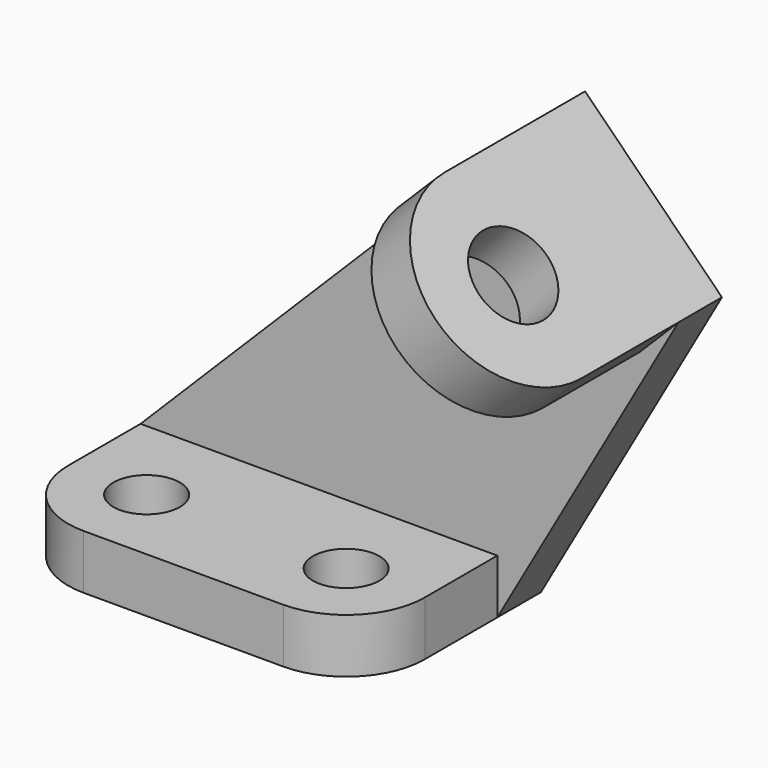
from build123d import *

# Parameters (mm, degrees)
F0_R     = 5.5
F1_DEPTH = 9
F2_DEPTH = 9
F4_DEPTH = 37
F5_DEPTH = 28
F6_R     = 7
F7_DEPTH = 9


with BuildPart() as f1:
    # F0 (on Top) → F1 (new body)
    with BuildSketch(Plane.XY):
        with BuildLine():
            ThreePointArc((-29.5, 13), (-25.6923881554, 3.8076118446), (-16.5, 0))
            Line((-16.5, 0), (16.5, 0))
            ThreePointArc((16.5, 0), (25.6923881554, 3.8076118446), (29.5, 13))
            Line((29.5, 13), (29.5, 37))
            Line((29.5, 37), (-29.5, 37))
            Line((-29.5, 37), (-29.5, 13))
        make_face()
        with Locations((-16.5, 13)):
            Circle(F0_R, mode=Mode.SUBTRACT)
        with Locations((16.5, 13)):
            Circle(F0_R, mode=Mode.SUBTRACT)
    extrude(amount=-F1_DEPTH)

    # F3 (on face) → F4 (join, through all)
    with BuildSketch(Plane.XZ):
        Polygon((36.813708499, 66.313708499), (25.5, 55), (48.127416998, 55), align=None)
        Polygon((48.127416998, 55), (25.5, 55), (-29.5, 0), (29.5, 0), (29.5, -9), (59.441125497, 43.686291501), align=None)
    extrude(amount=-F4_DEPTH)

    # F3 (on face) → F5 (cut)
    with BuildSketch(Plane.XZ):
        Polygon((36.813708499, 66.313708499), (25.5, 55), (48.127416998, 55), align=None)
        Polygon((48.127416998, 55), (25.5, 55), (-29.5, 0), (29.5, 0), (29.5, -9), (59.441125497, 43.686291501), align=None)
    extrude(amount=-F5_DEPTH, mode=Mode.SUBTRACT)

    # F6 (on face) → F7 (join)
    with BuildSketch(Plane(origin=(51.563708499, 0, 51.563708499), x_dir=(0.7071067812, 0, -0.7071067812), z_dir=(0.7071067812, 0, 0.7071067812))):
        with BuildLine():
            Line((11.140349955, 37), (-20.859650045, 37))
            Line((-20.859650045, 37), (-20.859650045, 8))
            ThreePointArc((-20.859650045, 8), (-4.859650045, -8), (11.140349955, 8))
            Line((11.140349955, 8), (11.140349955, 37))
        make_face()
        with Locations((-4.859650045, 8)):
            Circle(F6_R, mode=Mode.SUBTRACT)
    extrude(amount=-F7_DEPTH)


with BuildPart() as f2:
    # F0 (on Top) → F2 (new body)
    with BuildSketch(Plane.XY):
        with BuildLine():
            ThreePointArc((-29.5, 13), (-25.6923881554, 3.8076118446), (-16.5, 0))
            Line((-16.5, 0), (16.5, 0))
            ThreePointArc((16.5, 0), (25.6923881554, 3.8076118446), (29.5, 13))
            Line((29.5, 13), (29.5, 37))
            Line((29.5, 37), (-29.5, 37))
            Line((-29.5, 37), (-29.5, 13))
        make_face()
        with Locations((-16.5, 13)):
            Circle(F0_R, mode=Mode.SUBTRACT)
        with Locations((16.5, 13)):
            Circle(F0_R, mode=Mode.SUBTRACT)
    extrude(amount=-F2_DEPTH)


solid = Compound([f1.part, f2.part])
